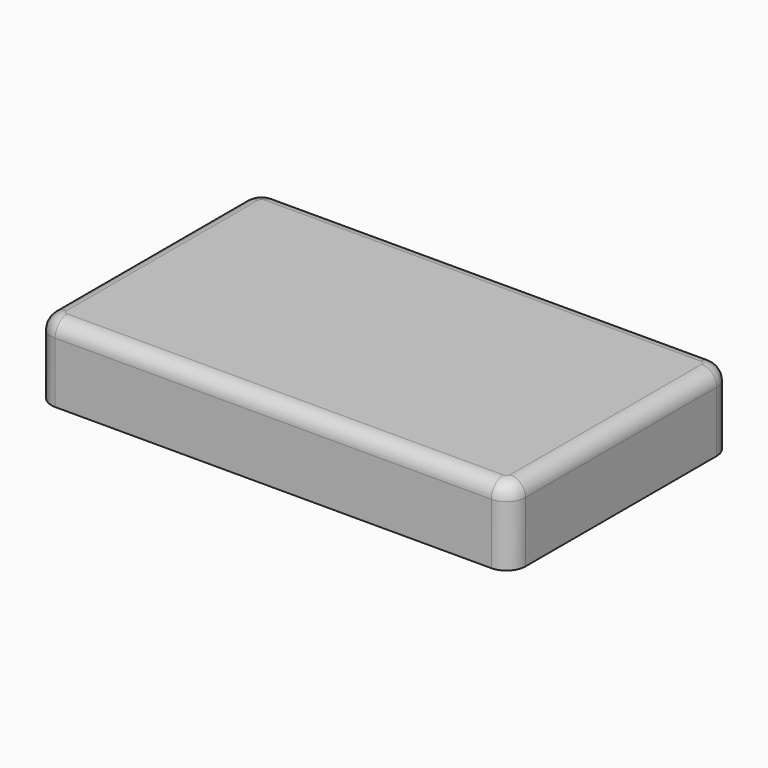
from build123d import *

# Parameters (mm, degrees)
F0_W         = 62.5
F0_H         = 36.5
F0_W_2       = 58.5
F0_H_2       = 31.5
F1_DEPTH     = 7
F3_DEPTH     = 1.5
F4_W         = 62.5
F4_H         = 36.5
F5_DEPTH     = 3
F7_DEPTH     = 2.5
F8_R         = 2.5
F9_T1_DEPTH  = 57.5
F9_T3_DEPTH  = 31.5
F9_T6_ANGLE  = 90
F9_T8_ANGLE  = 90
F9_T10_ANGLE = 90
F9_T12_ANGLE = 90
F10_W        = 1.25
F10_H        = 8.5
F11_DEPTH    = 2


# Not quite as in the source:
# - a fillet or chamfer that OpenCascade refuses, or shapes differently, is made with other operations: its cross-section is extruded or revolved along the edge and cut away or added


with BuildPart() as f1:
    # F0 (on Top) → F1 (new body)
    with BuildSketch(Plane.XY):
        with Locations((0.5, 0.5)):
            Rectangle(F0_W, F0_H)
        with Locations((1, 0.5)):
            Rectangle(F0_W_2, F0_H_2, mode=Mode.SUBTRACT)
    extrude(amount=F1_DEPTH)

    # F2 (on face) → F3 (join)
    with BuildSketch(Plane.XY.offset(7)):
        Polygon((30.25, 16.25), (-28.25, 16.25), (-28.25, -15.25), (30.25, -15.25), (30.25, -6), (30.25, 7), align=None)
    extrude(amount=-F3_DEPTH)

    # F4 (on face) → F5 (join)
    with BuildSketch(Plane(origin=(0, 0, 0), x_dir=(1, 0, 0), z_dir=(0, 0, -1))):
        with Locations((0.5, -0.5)):
            Rectangle(F4_W, F4_H)
        Polygon((-29.5, -17.522141248), (-29.5, 16.5), (30.25, 16.5), (30.25, 15.25), (30.25, -16.25), (30.25, -17.522141248), align=None, mode=Mode.SUBTRACT)
    extrude(amount=F5_DEPTH)

    # F6 (on face) → F7 (cut)
    with BuildSketch(Plane.YZ.offset(-28.25)):
        with BuildLine():
            Line((4, 5.5), (-3, 5.5))
            ThreePointArc((-3, 5.5), (-3.5303300859, 5.2803300859), (-3.75, 4.75))
            Line((-3.75, 4.75), (-3.75, 3.5))
            ThreePointArc((-3.75, 3.5), (-3.1642135624, 2.0857864376), (-1.75, 1.5))
            Line((-1.75, 1.5), (2.75, 1.5))
            ThreePointArc((2.75, 1.5), (4.1642135624, 2.0857864376), (4.75, 3.5))
            Line((4.75, 3.5), (4.75, 4.75))
            ThreePointArc((4.75, 4.75), (4.5303300859, 5.2803300859), (4, 5.5))
        make_face()
    extrude(amount=-F7_DEPTH, mode=Mode.SUBTRACT)

    # F8
    f8_edges = [f1.edges().sort_by_distance(p)[0] for p in [
        (-30.75, 18.75, 2),
        (-30.75, -17.75, 2),
        (31.75, 18.75, 2),
        (31.75, -17.75, 2),
    ]]
    fillet(f8_edges, radius=F8_R)

    # F9: fillet of radius 2 on 8 edges, made by hand

    # F9_s2 → F9_t1 (cut)
    with BuildSketch(Plane.YZ.offset(-28.25)):
        with BuildLine():
            ThreePointArc((-15.75, 7), (-17.1642135624, 6.4142135624), (-17.75, 5))
            Line((-17.75, 5), (-17.75, 7))
            Line((-17.75, 7), (-15.75, 7))
        make_face()
        with BuildLine():
            ThreePointArc((18.75, 5), (18.1642135624, 6.4142135624), (16.75, 7))
            Line((16.75, 7), (18.75, 7))
            Line((18.75, 7), (18.75, 5))
        make_face()
    extrude(amount=F9_T1_DEPTH, mode=Mode.SUBTRACT)

    # F9_s4 → F9_t3 (cut)
    with BuildSketch(Plane.XZ.offset(-16.25)):
        with BuildLine():
            ThreePointArc((29.75, 7), (31.1642135624, 6.4142135624), (31.75, 5))
            Line((31.75, 5), (31.75, 7))
            Line((31.75, 7), (29.75, 7))
        make_face()
        with BuildLine():
            ThreePointArc((-28.75, 7), (-30.1642135624, 6.4142135624), (-30.75, 5))
            Line((-30.75, 5), (-30.75, 7))
            Line((-30.75, 7), (-28.75, 7))
        make_face()
    extrude(amount=F9_T3_DEPTH, mode=Mode.SUBTRACT)

    # F9_s5 → F9_t6 (revolve, cut)
    with BuildSketch(Plane.YZ.offset(29.25)):
        with BuildLine():
            ThreePointArc((16.75, 7), (18.1642135624, 6.4142135624), (18.75, 5))
            Line((18.75, 5), (18.75, 7))
            Line((18.75, 7), (16.75, 7))
        make_face()
    revolve(axis=Axis((29.25, 16.25, 7), (0, 0, -1)), revolution_arc=F9_T6_ANGLE, mode=Mode.SUBTRACT)

    # F9_s7 → F9_t8 (revolve, cut)
    with BuildSketch(Plane.YZ.offset(-28.25)):
        with BuildLine():
            ThreePointArc((16.75, 7), (18.1642135624, 6.4142135624), (18.75, 5))
            Line((18.75, 5), (18.75, 7))
            Line((18.75, 7), (16.75, 7))
        make_face()
    revolve(axis=Axis((-28.25, 16.25, 7), (0, 0, 1)), revolution_arc=F9_T8_ANGLE, mode=Mode.SUBTRACT)

    # F9_s9 → F9_t10 (revolve, cut)
    with BuildSketch(Plane.XZ.offset(15.25)):
        with BuildLine():
            ThreePointArc((29.75, 7), (31.1642135624, 6.4142135624), (31.75, 5))
            Line((31.75, 5), (31.75, 7))
            Line((31.75, 7), (29.75, 7))
        make_face()
    revolve(axis=Axis((29.25, -15.25, 7), (0, 0, -1)), revolution_arc=F9_T10_ANGLE, mode=Mode.SUBTRACT)

    # F9_s11 → F9_t12 (revolve, cut)
    with BuildSketch(Plane.XZ.offset(15.25)):
        with BuildLine():
            ThreePointArc((-28.75, 7), (-30.1642135624, 6.4142135624), (-30.75, 5))
            Line((-30.75, 5), (-30.75, 7))
            Line((-30.75, 7), (-28.75, 7))
        make_face()
    revolve(axis=Axis((-28.25, -15.25, 7), (0, 0, 1)), revolution_arc=F9_T12_ANGLE, mode=Mode.SUBTRACT)

    # F10 (on face) → F11 (cut)
    with BuildSketch(Plane(origin=(0, 0, 0), x_dir=(1, 0, 0), z_dir=(0, 0, -1))):
        with Locations((-28.875, -0.5)):
            Rectangle(F10_W, F10_H)
    extrude(amount=-F11_DEPTH, mode=Mode.SUBTRACT)


solid = f1.part
